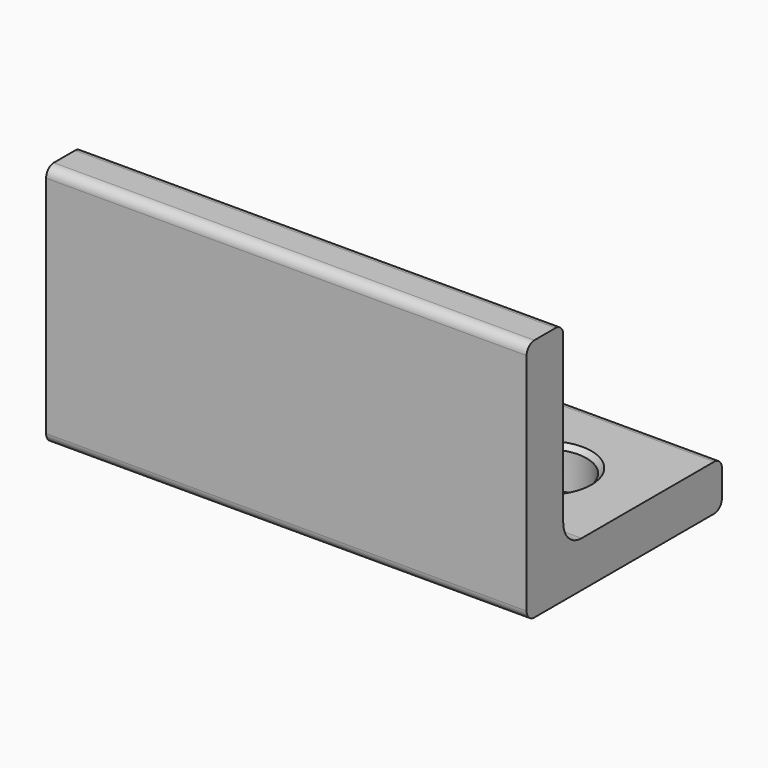
from build123d import *

# Parameters (mm, degrees)
F1_DEPTH = 25
F2_R     = 1
F3_R     = 2.38125
F4_R     = 4.25
F5_DEPTH = 25
F6_SIZE  = 0.5
F7_R     = 2.5
F8_DEPTH = 25


with BuildPart() as f1:
    # F0 (on Right) → F1 (new body, symmetric)
    with BuildSketch(Plane.YZ):
        Polygon((0, 25.4), (0, 0), (25.4, 0), (25.4, 4.7625), (4.7625, 4.7625), (4.7625, 25.4), align=None)
    extrude(amount=F1_DEPTH, both=True)

    # F2
    f2_edges = [f1.edges().sort_by_distance(p)[0] for p in [
        (0, 0, 25.4),
        (0, 4.7625, 25.4),
        (0, 0, 0),
        (0, 25.4, 4.7625),
        (0, 25.4, 0),
    ]]
    fillet(f2_edges, radius=F2_R)

    # F3
    f3_edges = [f1.edges().sort_by_distance(p)[0] for p in [
        (0, 4.7625, 4.7625),
    ]]
    fillet(f3_edges, radius=F3_R)

    # F4 (on face) → F5 (cut)
    with BuildSketch(Plane.XY.offset(4.7625)):
        with Locations((-15, 15)):
            Circle(F4_R)
        with Locations((715, 15)):
            Circle(F4_R)
        with Locations((1445, 15)):
            Circle(F4_R)
        with Locations((15, 15)):
            Circle(F4_R)
    extrude(amount=-F5_DEPTH, mode=Mode.SUBTRACT)

    # F6
    f6_edges = [f1.edges().sort_by_distance(p)[0] for p in [
        (-19.25, 15, 4.7625),
        (-10.75, 15, 2.38125),
        (-19.25, 15, 0),
        (10.75, 15, 4.7625),
        (19.25, 15, 2.38125),
        (10.75, 15, 0),
    ]]
    chamfer(f6_edges, length=F6_SIZE)

    # F7 (on face) → F8 (cut)
    with BuildSketch(Plane.XZ):
        with Locations((65, 20)):
            Circle(F7_R)
        with Locations((-65, 20)):
            Circle(F7_R)
    extrude(amount=-F8_DEPTH, mode=Mode.SUBTRACT)


solid = f1.part
